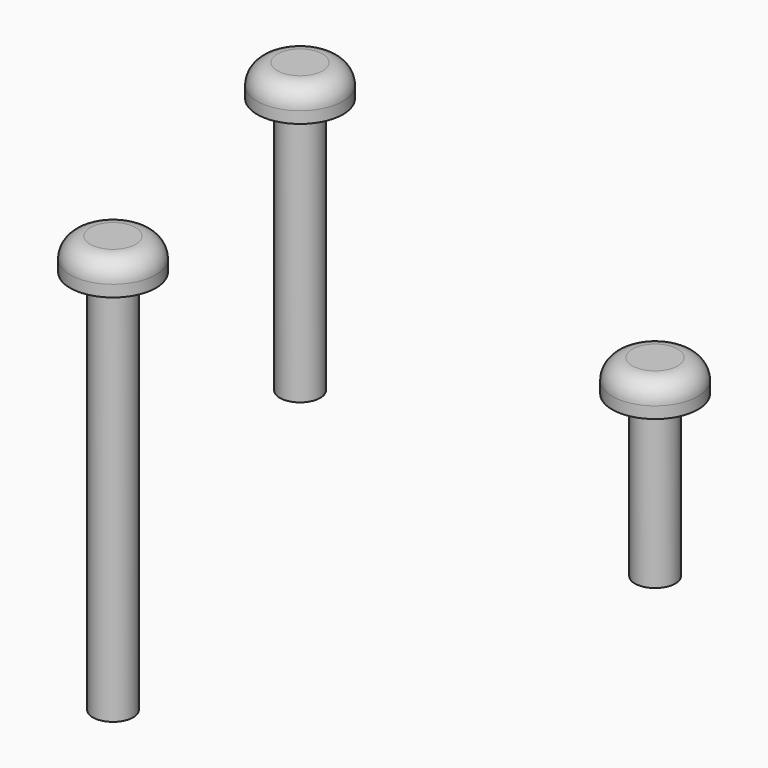
from build123d import *

# Parameters (mm, degrees)
F0_R     = 2.1209
F1_DEPTH = 1.5748
F2_R     = 1
F2_2_R   = 1
F2_3_R   = 1
F3_R     = 1
F4_DEPTH = 12.7
F5_R     = 1
F6_DEPTH = 19.05
F7_R     = 1
F8_DEPTH = 7.9375


# Not quite as in the source:
# - a length typed as a fraction of an inch, garbled in the dataset ("3 / 203.2 mm" for 3/8 in), is restored


with BuildPart() as f1:
    # F0 (on Top) → F1 (new body)
    with BuildSketch(Plane.XY):
        with Locations((-47.3690325885, 41.8840522646)):
            Circle(F0_R)
    extrude(amount=F1_DEPTH)

    # F2
    f2_edges = [f1.edges().sort_by_distance(p)[0] for p in [
        (-49.489933, 41.884052, 1.5748),
    ]]
    fillet(f2_edges, radius=F2_R)

    # F3 (on face) → F4 (join)
    with BuildSketch(Plane(origin=(0, 0, 0), x_dir=(1, 0, 0), z_dir=(0, 0, -1))):
        with Locations((-47.3690325885, -41.8840522646)):
            Circle(F3_R)
    extrude(amount=F4_DEPTH)


with BuildPart() as f1b:
    # F0 (on Top) → F1, piece 2 (new body)
    with BuildSketch(Plane.XY):
        with Locations((-43.9450238197, 26.0480039985)):
            Circle(F0_R)
    extrude(amount=F1_DEPTH)

    # F2#2
    f2_2_edges = [f1b.edges().sort_by_distance(p)[0] for p in [
        (-46.065924, 26.048004, 1.5748),
    ]]
    fillet(f2_2_edges, radius=F2_2_R)

    # F5 (on face) → F6 (join)
    with BuildSketch(Plane(origin=(0, 0, 0), x_dir=(1, 0, 0), z_dir=(0, 0, -1))):
        with Locations((-43.9450238197, -26.0480039985)):
            Circle(F5_R)
    extrude(amount=F6_DEPTH)


with BuildPart() as f1c:
    # F0 (on Top) → F1, piece 3 (new body)
    with BuildSketch(Plane.XY):
        with Locations((-21.260954018, 31.1840194363)):
            Circle(F0_R)
    extrude(amount=F1_DEPTH)

    # F2#3
    f2_3_edges = [f1c.edges().sort_by_distance(p)[0] for p in [
        (-23.381854, 31.184019, 1.5748),
    ]]
    fillet(f2_3_edges, radius=F2_3_R)

    # F7 (on face) → F8 (join)
    with BuildSketch(Plane(origin=(0, 0, 0), x_dir=(1, 0, 0), z_dir=(0, 0, -1))):
        with Locations((-21.260954018, -31.1840194363)):
            Circle(F7_R)
    extrude(amount=F8_DEPTH)


solid = Compound([f1.part, f1b.part, f1c.part])
